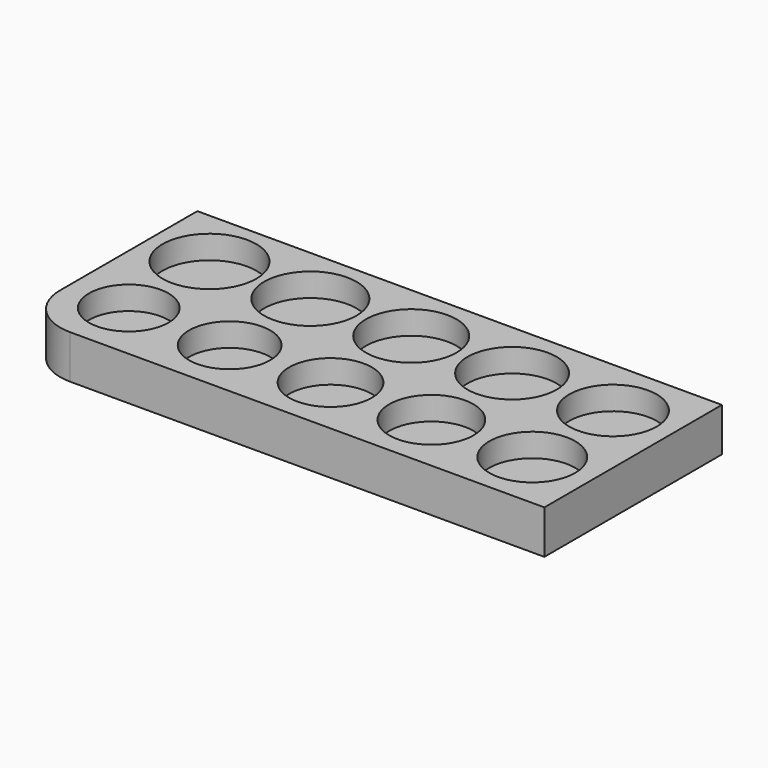
from build123d import *

# Parameters (mm, degrees)
F0_R     = 5.0038
F0_R_2   = 5.1038
F0_R_3   = 5.2038
F0_R_4   = 5.3038
F0_R_5   = 5.4038
F0_R_6   = 5.9038
F0_R_7   = 5.8038
F0_R_8   = 5.7038
F0_R_9   = 5.6038
F0_R_10  = 5.5038
F1_DEPTH = 2.9464
F2_R     = 5.9038
F2_R_2   = 5.8038
F2_R_3   = 5.7038
F2_R_4   = 5.6038
F2_R_5   = 5.5038
F2_R_6   = 5.0038
F2_R_7   = 5.1038
F2_R_8   = 5.2038
F2_R_9   = 5.3038
F2_R_10  = 5.4038
F3_DEPTH = 2.54


with BuildPart() as f1:
    # F0 (on Top) → F1 (new body)
    with BuildSketch(Plane.XY):
        with BuildLine():
            Line((27.8450359044, 20.32), (-38.1949640956, 20.32))
            Line((-38.1949640956, 20.32), (-38.1949640956, -1.27))
            ThreePointArc((-38.1949640956, -1.27), (-36.3350921561, -5.7601280605), (-31.8449640956, -7.62))
            Line((-31.8449640956, -7.62), (27.8450359044, -7.62))
            Line((27.8450359044, -7.62), (27.8450359044, 20.32))
        make_face()
        with Locations((-30.5749640956, 0)):
            Circle(F0_R, mode=Mode.SUBTRACT)
        with Locations((-17.8749640956, 0)):
            Circle(F0_R_2, mode=Mode.SUBTRACT)
        with Locations((-5.1749640956, 0)):
            Circle(F0_R_3, mode=Mode.SUBTRACT)
        with Locations((7.5250359044, 0)):
            Circle(F0_R_4, mode=Mode.SUBTRACT)
        with Locations((20.2250359044, 0)):
            Circle(F0_R_5, mode=Mode.SUBTRACT)
        with Locations((-30.5749640956, 12.7)):
            Circle(F0_R_6, mode=Mode.SUBTRACT)
        with Locations((-17.8749640956, 12.7)):
            Circle(F0_R_7, mode=Mode.SUBTRACT)
        with Locations((-5.1749640956, 12.7)):
            Circle(F0_R_8, mode=Mode.SUBTRACT)
        with Locations((7.5250359044, 12.7)):
            Circle(F0_R_9, mode=Mode.SUBTRACT)
        with Locations((20.2250359044, 12.7)):
            Circle(F0_R_10, mode=Mode.SUBTRACT)
    extrude(amount=F1_DEPTH)

    # F2 (on face) → F3 (join)
    with BuildSketch(Plane(origin=(0, 0, 0), x_dir=(1, 0, 0), z_dir=(0, 0, -1))):
        with BuildLine():
            Line((-38.1949640956, 1.27), (-38.1949640956, -20.32))
            Line((-38.1949640956, -20.32), (27.8450359044, -20.32))
            Line((27.8450359044, -20.32), (27.8450359044, 7.62))
            Line((27.8450359044, 7.62), (-31.8449640956, 7.62))
            ThreePointArc((-31.8449640956, 7.62), (-36.3350921561, 5.7601280605), (-38.1949640956, 1.27))
        make_face()
        with Locations((-30.5749640956, -12.7)):
            Circle(F2_R, mode=Mode.SUBTRACT)
        with Locations((-17.8749640956, -12.7)):
            Circle(F2_R_2, mode=Mode.SUBTRACT)
        with Locations((-5.1749640956, -12.7)):
            Circle(F2_R_3, mode=Mode.SUBTRACT)
        with Locations((7.5250359044, -12.7)):
            Circle(F2_R_4, mode=Mode.SUBTRACT)
        with Locations((20.2250359044, -12.7)):
            Circle(F2_R_5, mode=Mode.SUBTRACT)
        with Locations((-30.5749640956, 0)):
            Circle(F2_R_6, mode=Mode.SUBTRACT)
        with Locations((-17.8749640956, 0)):
            Circle(F2_R_7, mode=Mode.SUBTRACT)
        with Locations((-5.1749640956, 0)):
            Circle(F2_R_8, mode=Mode.SUBTRACT)
        with Locations((7.5250359044, 0)):
            Circle(F2_R_9, mode=Mode.SUBTRACT)
        with Locations((20.2250359044, 0)):
            Circle(F2_R_10, mode=Mode.SUBTRACT)
        with Locations((-30.5749640956, 0)):
            Circle(F2_R_6)
        with Locations((-30.5749640956, -12.7)):
            Circle(F2_R)
        with Locations((-17.8749640956, -12.7)):
            Circle(F2_R_2)
        with Locations((-17.8749640956, 0)):
            Circle(F2_R_7)
        with Locations((-5.1749640956, 0)):
            Circle(F2_R_8)
        with Locations((-5.1749640956, -12.7)):
            Circle(F2_R_3)
        with Locations((7.5250359044, -12.7)):
            Circle(F2_R_4)
        with Locations((7.5250359044, 0)):
            Circle(F2_R_9)
        with Locations((20.2250359044, 0)):
            Circle(F2_R_10)
        with Locations((20.2250359044, -12.7)):
            Circle(F2_R_5)
    extrude(amount=F3_DEPTH)


solid = f1.part
